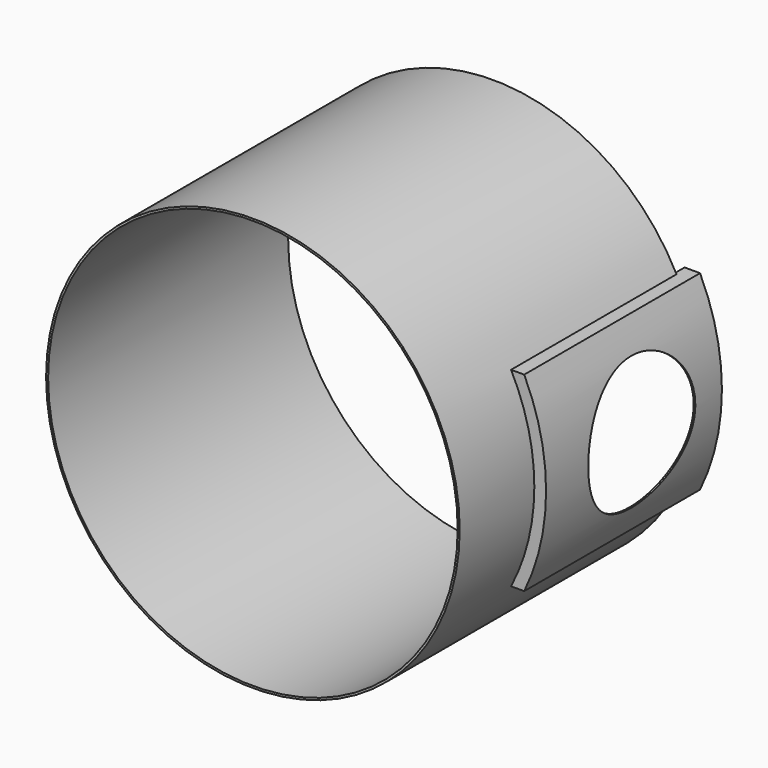
from build123d import *

# Parameters (mm, degrees)
F0_R        = 323.85
F0_R_2      = 320.675
F1_DEPTH    = 469.9
F2_W        = 298.45
F2_H        = 298.45
F3_DEPTH    = 595.884
F5_DEPTH    = 612.14
F6_T4_ANGLE = 57.0256517653
F7_R        = 669.2625565618
F7_R_2      = 339.725
F7_R_3      = 320.675
F8_DEPTH    = 561.34
F10_DEPTH   = 323.85
F11_R       = 104.775
F12_DEPTH   = 947.42
F13_DEPTH   = 20.32


# Not quite as in the source:
# - a fillet or chamfer that OpenCascade refuses, or shapes differently, is made with other operations: its cross-section is extruded or revolved along the edge and cut away or added


with BuildPart() as f1:
    # F0 (on Front) → F1 (new body)
    with BuildSketch(Plane.XZ):
        Circle(F0_R)
        Circle(F0_R_2, mode=Mode.SUBTRACT)
    extrude(amount=F1_DEPTH)

    # F2 (on Right) → F3 (cut)
    with BuildSketch(Plane.YZ):
        with Locations((-149.225, 0)):
            Rectangle(F2_W, F2_H)
    extrude(amount=F3_DEPTH, mode=Mode.SUBTRACT)

    # F4 (on Right) → F5 (join)
    with BuildSketch(Plane.YZ):
        Polygon((20.32, 149.225), (0, 149.225), (-323.85, 149.225), (-323.85, -149.225), (0, -149.225), (20.32, -149.225), (20.32, -144.145), (0, -144.145), (-17.1384390951, -144.145), (-306.7115609049, -144.145), (-306.7115609049, 144.145), (-17.1384390951, 144.145), (0, 144.145), (20.32, 144.145), align=None)
    extrude(amount=F5_DEPTH)

    # F6: fillet of radius 5.08 on 1 edges, made by hand


with BuildPart() as f6_tool2:
    # F6_s3 → F6_t4 (revolve)
    with BuildSketch(Plane(origin=(0, 0, 0), x_dir=(0, 1, 0), z_dir=(-0.4773554749, 0, 0.8787102768))):
        with BuildLine():
            ThreePointArc((-303.1592860393, -323.85), (-300.3194797079, -322.9821134838), (-298.45, -320.675))
            Line((-298.45, -320.675), (-298.45, -323.85))
            Line((-298.45, -323.85), (-303.1592860393, -323.85))
        make_face()
    revolve(axis=Axis((0, -298.45, 0), (0, 1, 0)), revolution_arc=F6_T4_ANGLE)

    split(bisect_by=Plane.XY.offset(-144.145), keep=Keep.TOP)

    split(bisect_by=Plane.XY.offset(144.145), keep=Keep.BOTTOM)


with BuildPart() as f1_1:
    add(f1.part)

    # F6_t1: cut F6_tool2
    add(f6_tool2.part, mode=Mode.SUBTRACT)

    # F7 (on Front) → F8 (cut, symmetric)
    with BuildSketch(Plane.XZ):
        Circle(F7_R)
        Circle(F7_R_2, mode=Mode.SUBTRACT)
        Circle(F7_R_3)
    extrude(amount=F8_DEPTH, both=True, mode=Mode.SUBTRACT)

    # F9 (on Front) → F10 (join, through all)
    with BuildSketch(Plane.XZ):
        with BuildLine():
            ThreePointArc((305.1966169537, 149.225), (339.725, 0), (305.1966169537, -149.225))
            Line((305.1966169537, -149.225), (308.0214758747, -149.225))
            ThreePointArc((308.0214758747, -149.225), (342.265, 0), (308.0214758747, 149.225))
            Line((308.0214758747, 149.225), (305.1966169537, 149.225))
        make_face()
    extrude(amount=F10_DEPTH)

    # F11 (on Right) → F12 (cut)
    with BuildSketch(Plane.YZ):
        with Locations((-136.525, 0)):
            Circle(F11_R)
    extrude(amount=F12_DEPTH, mode=Mode.SUBTRACT)

    # F9 (on Front) → F13 (join)
    with BuildSketch(Plane.XZ):
        with BuildLine():
            ThreePointArc((305.1966169537, 149.225), (339.725, 0), (305.1966169537, -149.225))
            Line((305.1966169537, -149.225), (308.0214758747, -149.225))
            ThreePointArc((308.0214758747, -149.225), (342.265, 0), (308.0214758747, 149.225))
            Line((308.0214758747, 149.225), (305.1966169537, 149.225))
        make_face()
    extrude(amount=-F13_DEPTH)


solid = f1_1.part
